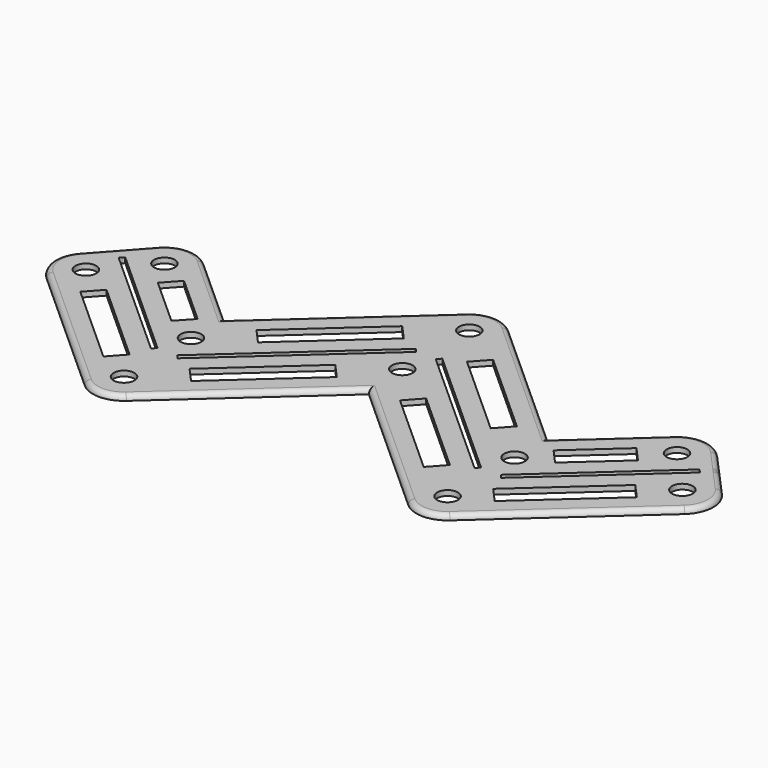
from build123d import *

# Parameters (mm, degrees)
F0_R     = 2
F1_DEPTH = 1
F2_R     = 0.99999


# Not quite as in the source:
# - a fillet or chamfer is up to 0.001 mm smaller than in the source, because OpenCascade refuses the exact size


with BuildPart() as f1:
    # F0 (on Top) → F1 (new body)
    with BuildSketch(Plane.XY):
        with BuildLine():
            Line((-56.070427214, 21.7097375971), (-58.2998616904, 23.7171294162))
            Line((-58.2998616904, 23.7171294162), (-61.9800800254, 19.6298328761))
            ThreePointArc((-61.9800800254, 19.6298328761), (-63.5129882811, 15.3010335004), (-61.5359947107, 11.156180285))
            Line((-61.5359947107, 11.156180285), (-35.2268663082, -12.5326653305))
            ThreePointArc((-35.2268663082, -12.5326653305), (-31.2120826701, -14.0737963776), (-27.1972990319, -12.5326653305))
            Line((-27.1972990319, -12.5326653305), (0, 11.9558927118))
            Line((0, 11.9558927118), (27.1972990319, -12.5326653305))
            ThreePointArc((27.1972990319, -12.5326653305), (31.2120826701, -14.0737963776), (35.2268663082, -12.5326653305))
            Line((35.2268663082, -12.5326653305), (61.5359947107, 11.156180285))
            ThreePointArc((61.5359947107, 11.156180285), (63.5129882811, 15.3010335004), (61.9800800254, 19.6298328761))
            Line((61.9800800254, 19.6298328761), (58.2998616904, 23.7171294162))
            Line((58.2998616904, 23.7171294162), (56.070427214, 21.7097375971))
            Line((56.070427214, 21.7097375971), (33.7760824497, 1.6358194063))
            Line((33.7760824497, 1.6358194063), (31.2120826701, -0.6728163648))
            Line((31.2120826701, -0.6728163648), (28.6480828904, 1.6358194063))
            Line((28.6480828904, 1.6358194063), (1.8948691733, 25.7245212353))
            Line((1.8948691733, 25.7245212353), (0, 27.4306691023))
            Line((0, 27.4306691023), (-1.8948691733, 25.7245212353))
            Line((-1.8948691733, 25.7245212353), (-28.6480828904, 1.6358194063))
            Line((-28.6480828904, 1.6358194063), (-31.2120826701, -0.6728163648))
            Line((-31.2120826701, -0.6728163648), (-33.7760824497, 1.6358194063))
            Line((-33.7760824497, 1.6358194063), (-56.070427214, 21.7097375971))
        make_face()
        with Locations((-31.2120826701, -8.0737963776)):
            Circle(F0_R, mode=Mode.SUBTRACT)
        Polygon((-53.6574585069, 9.4448453424), (-50.9809360815, 12.4174246443), (-35.0758352357, -1.9035924822), (-37.7523576611, -4.8761717841), align=None, mode=Mode.SUBTRACT)
        Polygon((-6.0931870421, 11.8520933749), (-22.4423732026, -2.868779965), (-25.118895628, 0.1037993369), (-8.7697094675, 14.8246726768), align=None, mode=Mode.SUBTRACT)
        with Locations((31.2120826701, -8.0737963776)):
            Circle(F0_R, mode=Mode.SUBTRACT)
        Polygon((22.4423732026, -2.868779965), (6.0931870421, 11.8520933749), (8.7697094675, 14.8246726768), (25.118895628, 0.1037993369), align=None, mode=Mode.SUBTRACT)
        Polygon((37.7523576611, -4.8761717841), (35.0758352357, -1.9035924822), (51.0113683193, 12.4448259544), (53.6878907447, 9.4722466525), align=None, mode=Mode.SUBTRACT)
        with Locations((-57.5212110725, 15.6150492379)):
            Circle(F0_R, mode=Mode.SUBTRACT)
        with Locations((0, 20.0296890894)):
            Circle(F0_R, mode=Mode.SUBTRACT)
        with Locations((57.5516433104, 15.6424505479)):
            Circle(F0_R, mode=Mode.SUBTRACT)
        Polygon((-55.7358619108, 22.0813100098), (-57.9652963872, 24.0887018289), (-58.2998616904, 23.7171294162), (-56.070427214, 21.7097375971), align=None)
        Polygon((-57.6307310841, 24.4602742417), (-57.9652963872, 24.0887018289), (-55.7358619108, 22.0813100098), (-55.4012966076, 22.4528824226), align=None)
        with BuildLine():
            Line((-53.9505127491, 28.5475707818), (-57.6307310841, 24.4602742417))
            Line((-57.6307310841, 24.4602742417), (-55.4012966076, 22.4528824226))
            Line((-55.4012966076, 22.4528824226), (-33.1069518433, 2.3789642318))
            Line((-33.1069518433, 2.3789642318), (-31.2120826701, 0.6728163648))
            Line((-31.2120826701, 0.6728163648), (-29.3172134968, 2.3789642318))
            Line((-29.3172134968, 2.3789642318), (-2.5639997796, 26.4676660607))
            Line((-2.5639997796, 26.4676660607), (0, 28.7763018319))
            Line((0, 28.7763018319), (2.5639997796, 26.4676660607))
            Line((2.5639997796, 26.4676660607), (29.3172134968, 2.3789642318))
            Line((29.3172134968, 2.3789642318), (31.2120826701, 0.6728163648))
            Line((31.2120826701, 0.6728163648), (33.1069518433, 2.3789642318))
            Line((33.1069518433, 2.3789642318), (55.4012966076, 22.4528824226))
            Line((55.4012966076, 22.4528824226), (57.6307310841, 24.4602742417))
            Line((57.6307310841, 24.4602742417), (53.9505127491, 28.5475707818))
            ThreePointArc((53.9505127491, 28.5475707818), (49.8056595337, 30.5245643522), (45.4768601581, 28.9916560965))
            Line((45.4768601581, 28.9916560965), (31.2120826701, 16.1475927553))
            Line((31.2120826701, 16.1475927553), (4.0147836382, 40.6361507976))
            ThreePointArc((4.0147836382, 40.6361507976), (0, 42.1772818447), (-4.0147836382, 40.6361507976))
            Line((-4.0147836382, 40.6361507976), (-31.2120826701, 16.1475927553))
            Line((-31.2120826701, 16.1475927553), (-45.4768601581, 28.9916560965))
            ThreePointArc((-45.4768601581, 28.9916560965), (-49.8056595337, 30.5245643522), (-53.9505127491, 28.5475707818))
        make_face()
        with Locations((-31.2120826701, 8.0737963776)):
            Circle(F0_R, mode=Mode.SUBTRACT)
        with Locations((31.2120826701, 8.0737963776)):
            Circle(F0_R, mode=Mode.SUBTRACT)
        Polygon((-46.3710360561, 19.0317138545), (-43.6945136306, 22.0042931564), (-34.3115040691, 13.5557933995), (-37.0313460748, 10.6222192229), align=None, mode=Mode.SUBTRACT)
        with Locations((-49.4916437962, 24.5327871436)):
            Circle(F0_R, mode=Mode.SUBTRACT)
        Polygon((-22.4423732026, 13.2788127903), (-25.118895628, 16.2513920922), (-8.7697094675, 30.9722654321), (-6.0931870421, 27.9996861302), align=None, mode=Mode.SUBTRACT)
        Polygon((6.0931870421, 27.9996861302), (8.7697094675, 30.9722654321), (25.118895628, 16.2513920922), (22.4423732026, 13.2788127903), align=None, mode=Mode.SUBTRACT)
        Polygon((37.0092128356, 10.6022903648), (34.3326904102, 13.5748696667), (43.6361429708, 21.9517359782), (46.3126653962, 18.9791566763), align=None, mode=Mode.SUBTRACT)
        with Locations((49.4332731364, 24.4802299654)):
            Circle(F0_R, mode=Mode.SUBTRACT)
        with Locations((0, 36.1772818447)):
            Circle(F0_R, mode=Mode.SUBTRACT)
        Polygon((-31.2120826701, 0), (-33.4415171465, 2.0073918191), (-33.7760824497, 1.6358194063), (-31.2120826701, -0.6728163648), (-28.6480828904, 1.6358194063), (-28.9826481936, 2.0073918191), align=None)
        Polygon((-33.1069518433, 2.3789642318), (-33.4415171465, 2.0073918191), (-31.2120826701, 0), (-28.9826481936, 2.0073918191), (-29.3172134968, 2.3789642318), (-31.2120826701, 0.6728163648), align=None)
        Polygon((0, 28.1034854671), (-2.2294344764, 26.096093648), (-1.8948691733, 25.7245212353), (0, 27.4306691023), (1.8948691733, 25.7245212353), (2.2294344764, 26.096093648), align=None)
        Polygon((-2.5639997796, 26.4676660607), (-2.2294344764, 26.096093648), (0, 28.1034854671), (2.2294344764, 26.096093648), (2.5639997796, 26.4676660607), (0, 28.7763018319), align=None)
        Polygon((31.2120826701, 0), (28.9826481936, 2.0073918191), (28.6480828904, 1.6358194063), (31.2120826701, -0.6728163648), (33.7760824497, 1.6358194063), (33.4415171465, 2.0073918191), align=None)
        Polygon((29.3172134968, 2.3789642318), (28.9826481936, 2.0073918191), (31.2120826701, 0), (33.4415171465, 2.0073918191), (33.1069518433, 2.3789642318), (31.2120826701, 0.6728163648), align=None)
        Polygon((57.9652963872, 24.0887018289), (55.7358619108, 22.0813100098), (56.070427214, 21.7097375971), (58.2998616904, 23.7171294162), align=None)
        Polygon((57.9652963872, 24.0887018289), (57.6307310841, 24.4602742417), (55.4012966076, 22.4528824226), (55.7358619108, 22.0813100098), align=None)
    extrude(amount=F1_DEPTH)

    # F2 (radius 1 in the source; OpenCascade refuses exactly that, so slightly less here)
    f2_edges = [f1.edges().sort_by_distance(p)[0] for p in [
        (-63.512988, 15.301034, 1),
        (-48.381431, -0.688243, 1),
        (-31.212083, -14.073796, 1),
        (-13.59865, -0.288386, 1),
        (13.59865, -0.288386, 1),
        (31.212083, -14.073796, 1),
        (48.381431, -0.688243, 1),
        (63.512988, 15.301034, 1),
        (57.965296, 24.088702, 1),
        (49.80566, 30.524564, 1),
        (38.344471, 22.569624, 1),
        (17.613433, 28.391872, 1),
        (0, 42.177282, 1),
        (-17.613433, 28.391872, 1),
        (-38.344471, 22.569624, 1),
        (-49.80566, 30.524564, 1),
        (-57.965296, 24.088702, 1),
    ]]
    fillet(f2_edges, radius=F2_R)


solid = f1.part
